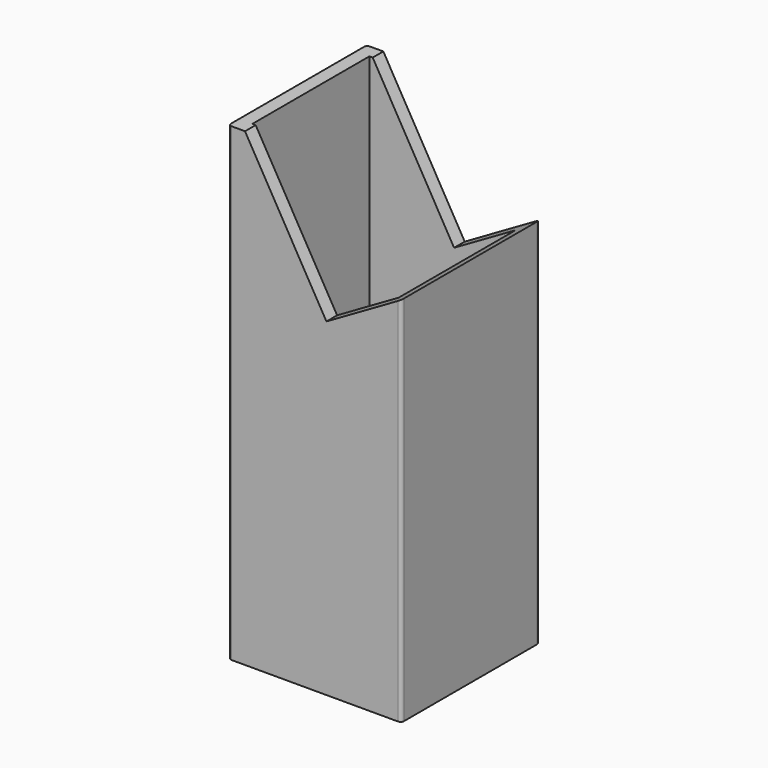
from build123d import *

# Parameters (mm, degrees)
F0_W     = 26
F0_H     = 26
F0_W_2   = 22
F0_H_2   = 22
F1_DEPTH = 75
F3_DEPTH = 26.001
F4_R     = 0.5


# Not quite as in the source:
# - a feature names something its author has since deleted; it is built from what else it names


with BuildPart() as f1:
    # F0 (on Top) → F1 (new body)
    with BuildSketch(Plane.XY):
        Rectangle(F0_W, F0_H)
        Rectangle(F0_W_2, F0_H_2, mode=Mode.SUBTRACT)
    extrude(amount=F1_DEPTH)

    # F2 (on face) → F3 (cut, through all)
    with BuildSketch(Plane(origin=(0, 13, 0), x_dir=(-1, 0, 0), z_dir=(0, 1, 0))):
        Polygon((-13, 55.9666790032), (-1.7416697508, 49.4666790032), (10.5, 70.6698729811), (13, 70.6698729811), (13, 75), (-8.7376814767, 75), (-13, 75), align=None)
    extrude(amount=-F3_DEPTH, mode=Mode.SUBTRACT)

    # F4
    f4_edges = [f1.edges().sort_by_distance(p)[0] for p in [
        (13, 13, 27.98334),
        (-13, 13, 35.334936),
        (-13, -13, 35.334936),
        (13, -13, 27.98334),
    ]]
    fillet(f4_edges, radius=F4_R)


solid = f1.part
